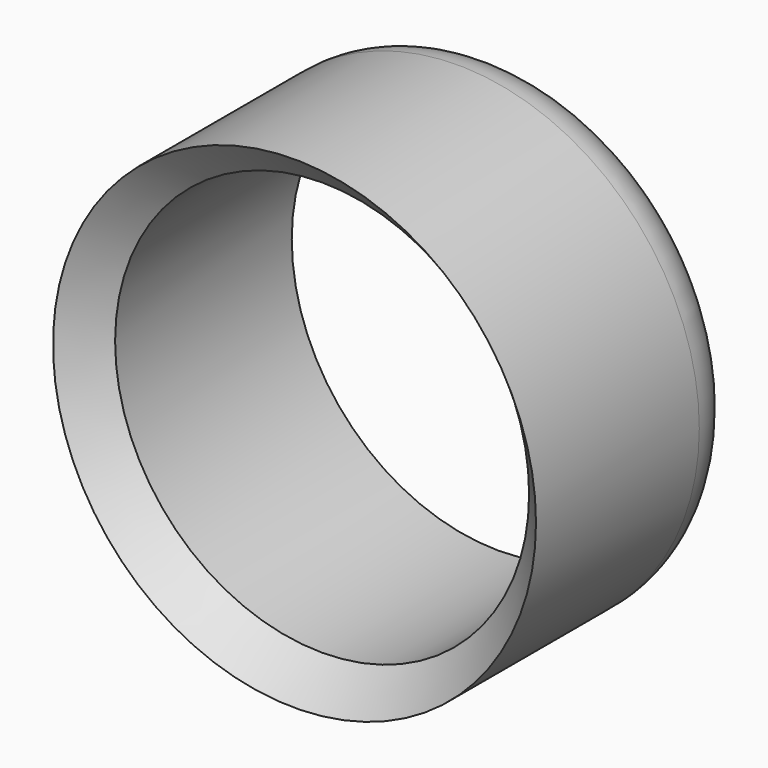
from build123d import *

# Parameters (mm, degrees)
F0_R     = 22.225
F1_DEPTH = 25.4
F2_T     = -3.175


# Not quite as in the source:
# - a fillet or chamfer that OpenCascade refuses, or shapes differently, is made with other operations: its cross-section is extruded or revolved along the edge and cut away or added


with BuildPart() as f1:
    # F0 (on Front) → F1 (new body)
    with BuildSketch(Plane.XZ):
        Circle(F0_R)
    extrude(amount=-F1_DEPTH)

    # F2
    f2_openings = [f1.faces().sort_by_distance(p)[0] for p in [
        (0, 0, 0),
        (0, 25.4, 0),
    ]]
    offset(amount=F2_T, openings=f2_openings)

    # F3: chamfer of 5.08 on 1 edges, made by hand

    # F3_s1 → F3_t2 (revolve, cut)
    with BuildSketch(Plane.XY):
        Polygon((24.13, 0), (19.05, 5.08), (19.05, 0), align=None)
    revolve(axis=Axis((0, 0, 0), (0, -1, 0)), mode=Mode.SUBTRACT)

    # F4: fillet of radius 5.08 on 1 edges, made by hand

    # F4_s1 → F4_t2 (revolve, cut)
    with BuildSketch(Plane.XY):
        with BuildLine():
            ThreePointArc((22.225, 20.6907139607), (21.3571134838, 23.5305202921), (19.05, 25.4))
            Line((19.05, 25.4), (22.225, 25.4))
            Line((22.225, 25.4), (22.225, 20.6907139607))
        make_face()
    revolve(axis=Axis((0, 25.4, 0), (0, -1, 0)), mode=Mode.SUBTRACT)


solid = f1.part
